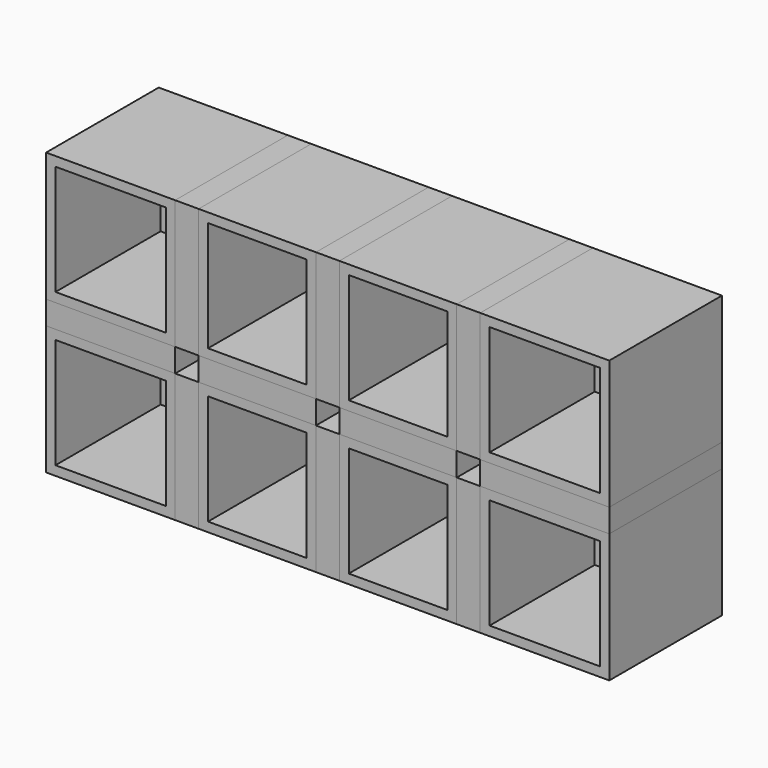
from build123d import *

# Parameters (mm, degrees)
F0_W     = 34.925
F0_H     = 34.925
F1_DEPTH = 38.1
F0_W_2   = 31.75
F2_T     = -2.54
F2_2_T   = -2.54
F2_3_T   = -2.54
F2_4_T   = -2.54
F2_5_T   = -2.54
F2_6_T   = -2.54
F2_7_T   = -2.54
F2_8_T   = -2.54
F0_H_2   = 6.35
F3_DEPTH = 38.1
F0_W_3   = 6.35


with BuildPart() as f1:
    # F0 (on Front) → F1 (new body)
    with BuildSketch(Plane.XZ):
        with Locations((-58.7375, 20.6375)):
            Rectangle(F0_W, F0_H)
    extrude(amount=-F1_DEPTH)

    # F2
    f2_openings = [f1.faces().sort_by_distance(p)[0] for p in [
        (-58.7375, 0, 20.6375),
    ]]
    offset(amount=F2_T, openings=f2_openings)


with BuildPart() as f1b:
    # F0 (on Front) → F1, piece 2 (new body)
    with BuildSketch(Plane.XZ):
        with Locations((-19.05, 20.6375)):
            Rectangle(F0_W_2, F0_H)
    extrude(amount=-F1_DEPTH)

    # F2#2
    f2_2_openings = [f1b.faces().sort_by_distance(p)[0] for p in [
        (-19.05, 0, 20.6375),
    ]]
    offset(amount=F2_2_T, openings=f2_2_openings)


with BuildPart() as f1c:
    # F0 (on Front) → F1, piece 3 (new body)
    with BuildSketch(Plane.XZ):
        with Locations((19.05, 20.6375)):
            Rectangle(F0_W_2, F0_H)
    extrude(amount=-F1_DEPTH)

    # F2#3
    f2_3_openings = [f1c.faces().sort_by_distance(p)[0] for p in [
        (19.05, 0, 20.6375),
    ]]
    offset(amount=F2_3_T, openings=f2_3_openings)


with BuildPart() as f1d:
    # F0 (on Front) → F1, piece 4 (new body)
    with BuildSketch(Plane.XZ):
        with Locations((58.7375, 20.6375)):
            Rectangle(F0_W, F0_H)
    extrude(amount=-F1_DEPTH)

    # F2#4
    f2_4_openings = [f1d.faces().sort_by_distance(p)[0] for p in [
        (58.7375, 0, 20.6375),
    ]]
    offset(amount=F2_4_T, openings=f2_4_openings)


with BuildPart() as f1e:
    # F0 (on Front) → F1, piece 5 (new body)
    with BuildSketch(Plane.XZ):
        with Locations((58.7375, -20.6375)):
            Rectangle(F0_W, F0_H)
    extrude(amount=-F1_DEPTH)

    # F2#5
    f2_5_openings = [f1e.faces().sort_by_distance(p)[0] for p in [
        (58.7375, 0, -20.6375),
    ]]
    offset(amount=F2_5_T, openings=f2_5_openings)


with BuildPart() as f1f:
    # F0 (on Front) → F1, piece 6 (new body)
    with BuildSketch(Plane.XZ):
        with Locations((19.05, -20.6375)):
            Rectangle(F0_W_2, F0_H)
    extrude(amount=-F1_DEPTH)

    # F2#6
    f2_6_openings = [f1f.faces().sort_by_distance(p)[0] for p in [
        (19.05, 0, -20.6375),
    ]]
    offset(amount=F2_6_T, openings=f2_6_openings)


with BuildPart() as f1g:
    # F0 (on Front) → F1, piece 7 (new body)
    with BuildSketch(Plane.XZ):
        with Locations((-19.05, -20.6375)):
            Rectangle(F0_W_2, F0_H)
    extrude(amount=-F1_DEPTH)

    # F2#7
    f2_7_openings = [f1g.faces().sort_by_distance(p)[0] for p in [
        (-19.05, 0, -20.6375),
    ]]
    offset(amount=F2_7_T, openings=f2_7_openings)


with BuildPart() as f1h:
    # F0 (on Front) → F1, piece 8 (new body)
    with BuildSketch(Plane.XZ):
        with Locations((-58.7375, -20.6375)):
            Rectangle(F0_W, F0_H)
    extrude(amount=-F1_DEPTH)

    # F2#8
    f2_8_openings = [f1h.faces().sort_by_distance(p)[0] for p in [
        (-58.7375, 0, -20.6375),
    ]]
    offset(amount=F2_8_T, openings=f2_8_openings)


with BuildPart() as f3:
    # F0 (on Front) → F3 (new body)
    with BuildSketch(Plane.XZ):
        with Locations((-58.7375, 0)):
            Rectangle(F0_W, F0_H_2)
    extrude(amount=-F3_DEPTH)


with BuildPart() as f3b:
    # F0 (on Front) → F3, piece 2 (new body)
    with BuildSketch(Plane.XZ):
        Polygon((-34.925, 3.175), (-34.925, 38.1), (-38.1, 38.1), (-41.275, 38.1), (-41.275, 3.175), align=None)
    extrude(amount=-F3_DEPTH)


with BuildPart() as f3c:
    # F0 (on Front) → F3, piece 3 (new body)
    with BuildSketch(Plane.XZ):
        with Locations((-19.05, 0)):
            Rectangle(F0_W_2, F0_H_2)
    extrude(amount=-F3_DEPTH)


with BuildPart() as f3d:
    # F0 (on Front) → F3, piece 4 (new body)
    with BuildSketch(Plane.XZ):
        Polygon((-34.925, -38.1), (-34.925, -3.175), (-41.275, -3.175), (-41.275, -38.1), (-38.1, -38.1), align=None)
    extrude(amount=-F3_DEPTH)


with BuildPart() as f3e:
    # F0 (on Front) → F3, piece 5 (new body)
    with BuildSketch(Plane.XZ):
        with Locations((0, -20.6375)):
            Rectangle(F0_W_3, F0_H)
    extrude(amount=-F3_DEPTH)


with BuildPart() as f3f:
    # F0 (on Front) → F3, piece 6 (new body)
    with BuildSketch(Plane.XZ):
        with Locations((0, 20.6375)):
            Rectangle(F0_W_3, F0_H)
    extrude(amount=-F3_DEPTH)


with BuildPart() as f3g:
    # F0 (on Front) → F3, piece 7 (new body)
    with BuildSketch(Plane.XZ):
        Polygon((41.275, 3.175), (41.275, 38.1), (38.1, 38.1), (34.925, 38.1), (34.925, 3.175), align=None)
    extrude(amount=-F3_DEPTH)


with BuildPart() as f3h:
    # F0 (on Front) → F3, piece 8 (new body)
    with BuildSketch(Plane.XZ):
        Polygon((41.275, -38.1), (41.275, -3.175), (34.925, -3.175), (34.925, -38.1), (38.1, -38.1), align=None)
    extrude(amount=-F3_DEPTH)


with BuildPart() as f3i:
    # F0 (on Front) → F3, piece 9 (new body)
    with BuildSketch(Plane.XZ):
        with Locations((58.7375, 0)):
            Rectangle(F0_W, F0_H_2)
    extrude(amount=-F3_DEPTH)


with BuildPart() as f3j:
    # F0 (on Front) → F3, piece 10 (new body)
    with BuildSketch(Plane.XZ):
        with Locations((19.05, 0)):
            Rectangle(F0_W_2, F0_H_2)
    extrude(amount=-F3_DEPTH)


solid = Compound([f1.part, f1b.part, f1c.part, f1d.part, f1e.part, f1f.part, f1g.part, f1h.part, f3.part, f3b.part, f3c.part, f3d.part, f3e.part, f3f.part, f3g.part, f3h.part, f3i.part, f3j.part])
